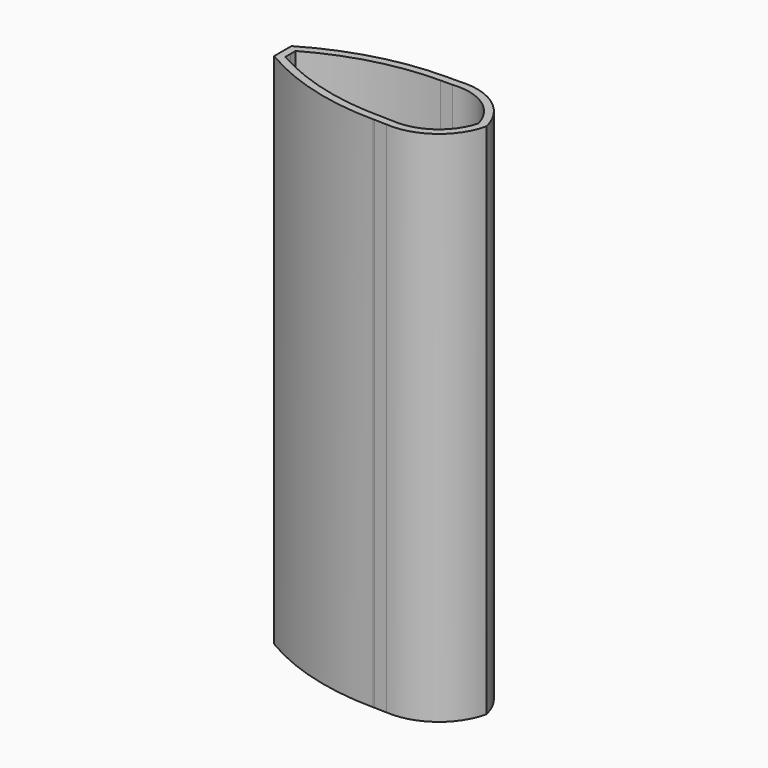
from build123d import *

# Parameters (mm, degrees)
F1_DEPTH = 168


# Not quite as in the source:
# - a feature names something its author has since deleted; it is built from what else it names


with BuildPart() as f1:
    # F0 (on Top) → F1 (new body)
    with BuildSketch(Plane.XY):
        with BuildLine():
            add(Edge.make_bspline(
                [(9.0589725163, 14.9090803276), (9.1893761129, 14.9089854783), (9.3201289556, 14.9089586218), (9.4512325362, 14.909)],
                knots=[108.3727376298, 108.3727376298, 108.3727376298, 108.3727376298, 108.6044995707, 108.6044995707, 108.6044995707, 108.6044995707], degree=3))
            ThreePointArc((9.0589725163, 14.9090803276), (-12.3350874174, 11.9828700727), (-32.1953748348, 3.5071700662))
            Line((-32.1953748348, 3.5071700662), (-32.1954637008, 6.33471e-05))
            Line((-32.1954637008, 6.33471e-05), (-32.1955525689, -3.5071262621))
            ThreePointArc((-32.1955525689, -3.5071262621), (-12.3352527385, -11.9828512354), (9.0588260182, -14.9090804342))
            add(Edge.make_bspline(
                [(9.0588260182, -14.9090804342), (9.1892781859, -14.9089854984), (9.3200798608, -14.9089586063), (9.4512325362, -14.909)],
                knots=[108.372650841, 108.372650841, 108.372650841, 108.372650841, 108.6044995707, 108.6044995707, 108.6044995707, 108.6044995707], degree=3))
            Line((9.4512325362, -14.909), (13.4156349212, -15.0296401869))
            ThreePointArc((13.4156349212, -15.0296401869), (26.4575983511, -11.3147653424), (33.9237386916, 0.0055638769))
            ThreePointArc((33.9237386916, 0.0055638769), (26.221744338, 11.4277863656), (12.8924894738, 14.909))
            Line((12.8924894738, 14.909), (9.4512325362, 14.909))
        make_face()
        with BuildLine():
            Line((-29.6955161871, -2.0713442572), (-29.6954637016, 0))
            Line((-29.6954637016, 0), (-29.6954112161, 2.0713449993))
            ThreePointArc((-29.6954112161, 2.0713449993), (-11.0041823718, 9.7538427825), (9.0291136139, 12.409))
            Line((9.0291136139, 12.409), (13.0291136139, 12.409))
            ThreePointArc((13.0291136139, 12.409), (24.4821941123, 9.5918072896), (31.3456378974, 0))
            ThreePointArc((31.3456378974, 0), (24.7175372439, -9.4867852182), (13.5527042793, -12.5326540468))
            Line((13.5527042793, -12.5326540468), (4.2194331318, -12.2486345488))
            ThreePointArc((4.2194331318, -12.2486345488), (-13.3194868099, -9.0976060688), (-29.6955161871, -2.0713442572))
        make_face(mode=Mode.SUBTRACT)
    extrude(amount=-F1_DEPTH)


solid = f1.part
